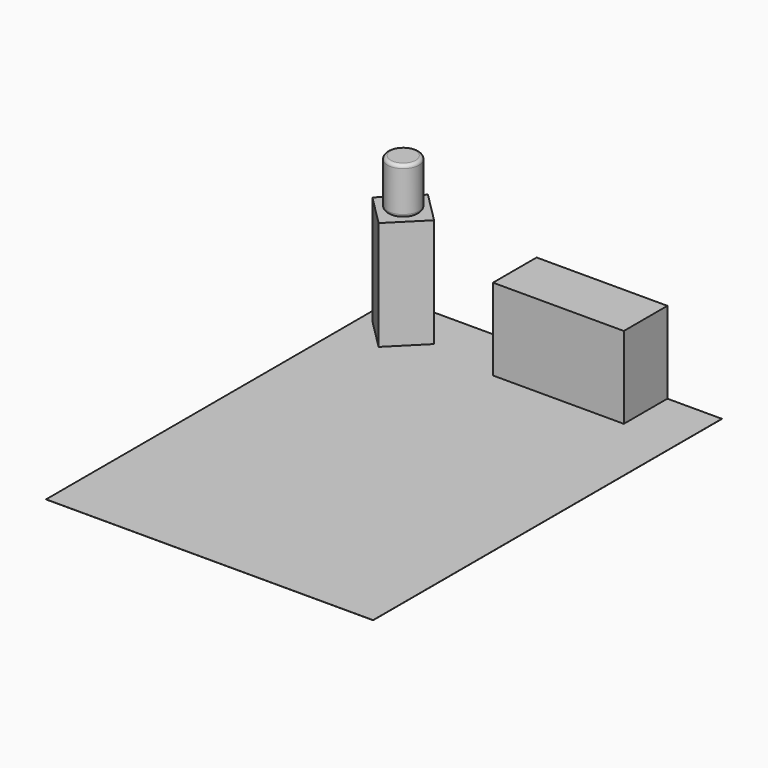
from build123d import *

# Parameters (mm, degrees)
F0_W     = 3000
F0_H     = 4000
F2_DEPTH = 1
F5_DEPTH = 1000
F3_W     = 1200
F3_H     = 500
F6_DEPTH = 750


# Not quite as in the source:
# - the program builds the solid bodies; features that only make, move or delete a surface that nothing else refers to are left out


with BuildPart() as f2:
    # F0 (on Top) → F2 (new body)
    with BuildSketch(Plane.XY):
        with Locations((1500, 2000)):
            Rectangle(F0_W, F0_H)
    extrude(amount=-F2_DEPTH)

    # F4 (on Top) → F5 (join)
    with BuildSketch(Plane.XY):
        Polygon((665.6854249492, 3617.1572875254), (382.8427124746, 3900), (100, 3617.1572875254), (382.8427124746, 3334.3145750508), align=None)
    extrude(amount=F5_DEPTH)

    # F3 (on face) → F6 (join)
    with BuildSketch(Plane.XY):
        with Locations((1900, 3750)):
            Rectangle(F3_W, F3_H)
    extrude(amount=F6_DEPTH)

    # F8 (on offset) → F9 (revolve)
    with BuildSketch(Plane(origin=(-1617.1572875254, 1617.1572875254, 0), x_dir=(0.7071067812, 0.7071067812, 0), z_dir=(0.7071067812, -0.7071067812, 0))):
        with BuildLine():
            Line((2803.4271247462, 900), (2828.4271247462, 900))
            Line((2828.4271247462, 900), (2828.4271247462, 1430))
            Line((2828.4271247462, 1430), (2713.4271247462, 1430))
            ThreePointArc((2713.4271247462, 1430), (2692.2139213106, 1421.2132034356), (2683.4271247462, 1400))
            Line((2683.4271247462, 1400), (2683.4271247462, 1030))
            ThreePointArc((2683.4271247462, 1030), (2692.2139213106, 1008.7867965644), (2713.4271247462, 1000))
            Line((2713.4271247462, 1000), (2803.4271247462, 1000))
            Line((2803.4271247462, 1000), (2803.4271247462, 900))
        make_face()
    revolve(axis=Axis((382.8427124746, 3617.1572875254, 1165), (0, 0, 1)))


solid = f2.part
